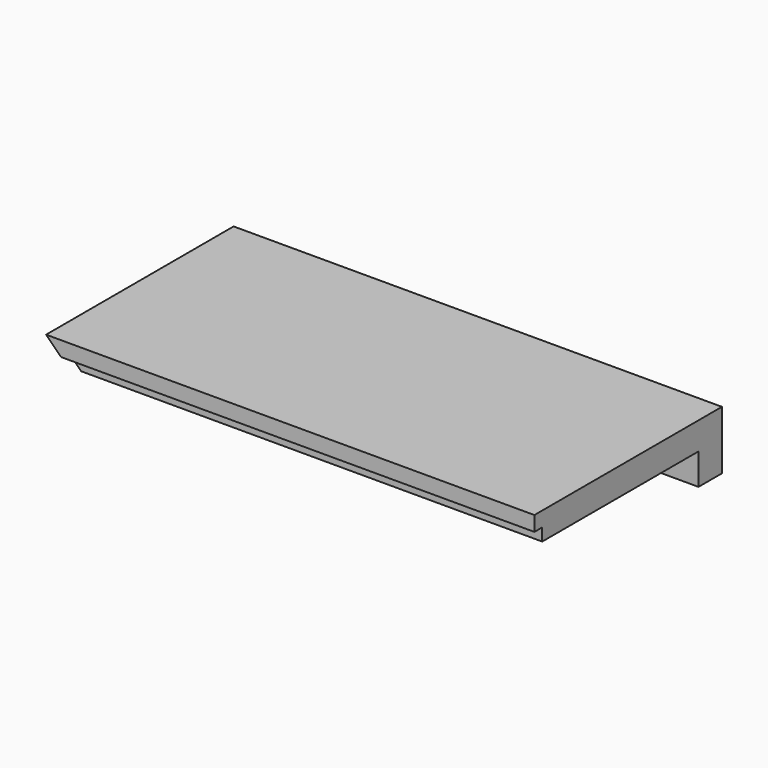
from build123d import *

# Parameters (mm, degrees)
F1_DEPTH = 76.2
F2_W     = 153.924
F2_H     = 153.924
F3_DEPTH = 3.175
F4_W     = 149.86
F4_H     = 149.86
F5_DEPTH = 63.5
F7_DEPTH = 76.201


# Not quite as in the source:
# - a feature names something its author has since deleted; it is built from what else it names


with BuildPart() as f1:
    # F0 (on Front) → F1 (new body)
    with BuildSketch(Plane.XZ):
        Polygon((0, 139.7), (0, 158.75), (-158.75, 158.75), (-158.75, 0), (-139.7, 0), (-139.7, 139.7), align=None)
    extrude(amount=F1_DEPTH)

    # F2 (on face) → F3 (cut)
    with BuildSketch(Plane.XZ.offset(76.2)):
        with Locations((-76.962, 76.962)):
            Rectangle(F2_W, F2_H)
    extrude(amount=-F3_DEPTH, mode=Mode.SUBTRACT)

    # F4 (on face) → F5 (cut)
    with BuildSketch(Plane.XZ.offset(73.025)):
        with Locations((-74.93, 74.93)):
            Rectangle(F4_W, F4_H)
    extrude(amount=-F5_DEPTH, mode=Mode.SUBTRACT)

    # F6 (on face) → F7 (cut, through all)
    with BuildSketch(Plane.XZ.offset(76.2)):
        Polygon((-139.7, 139.7), (-158.75, 158.75), (-158.75, 0), (-139.7, 0), align=None)
    extrude(amount=-F7_DEPTH, mode=Mode.SUBTRACT)


solid = f1.part
